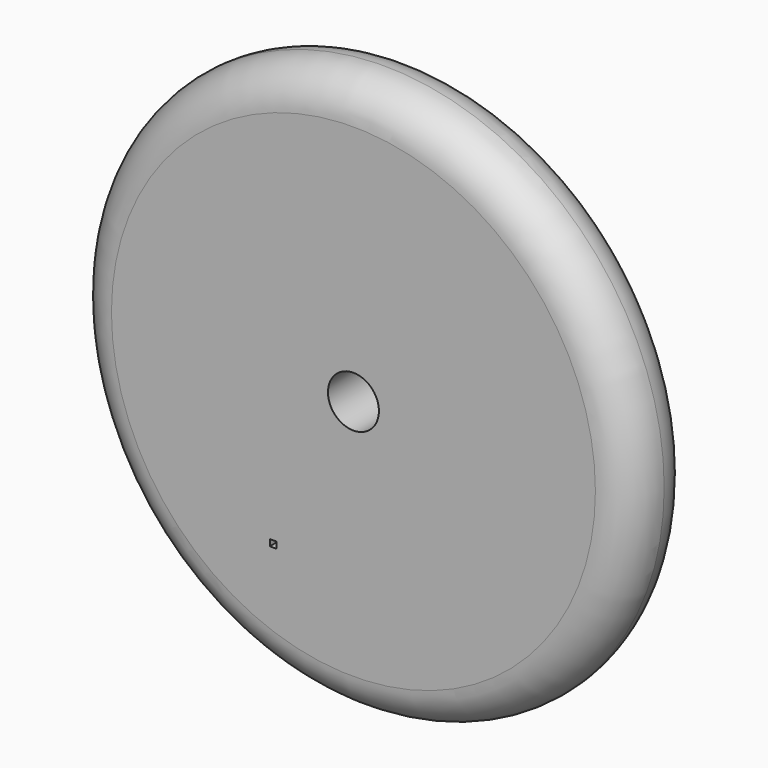
from build123d import *

# Parameters (mm, degrees)
F0_R     = 6.985
F0_W     = 0.1642033458
F0_H     = 0.1596324146
F0_R_2   = 0.635
F1_DEPTH = 1.905
F2_R     = 0.95249


# Not quite as in the source:
# - a fillet or chamfer is up to 0.001 mm smaller than in the source, because OpenCascade refuses the exact size


with BuildPart() as f1:
    # F0 (on Front) → F1 (new body)
    with BuildSketch(Plane.XZ):
        with Locations((-56.4259625971, 38.3895114064)):
            Circle(F0_R)
        with Locations((-58.4293603897, 34.6161220223)):
            Rectangle(F0_W, F0_H, mode=Mode.SUBTRACT)
        with Locations((-56.4259625971, 38.3895114064)):
            Circle(F0_R_2, mode=Mode.SUBTRACT)
    extrude(amount=F1_DEPTH)

    # F2 (radius 0.9525 in the source; OpenCascade refuses exactly that, so slightly less here)
    f2_edges = [f1.edges().sort_by_distance(p)[0] for p in [
        (-63.410963, -1.905, 38.389511),
        (-63.410963, 0, 38.389511),
    ]]
    fillet(f2_edges, radius=F2_R)


solid = f1.part
